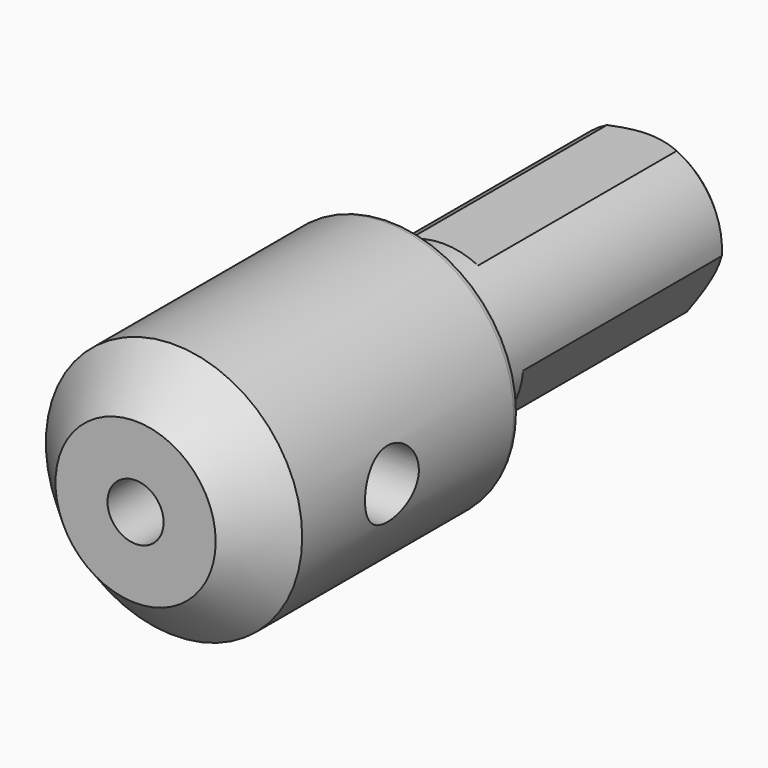
from build123d import *

# Parameters (mm, degrees)
F0_R            = 8
F1_DEPTH        = 20
F2_R            = 5
F3_DEPTH        = 20
F5_DEPTH        = 16
F5_COPIES_COUNT = 3
F6_SIZE         = 0.49999
F7_R            = 0.5
F9_D            = 3.5
F9_DEPTH        = 14
F9_TIP          = 1.0515060833
F10_R           = 2.1
F11_DEPTH       = 8.25
F12_SIZE        = 3


# Not quite as in the source:
# - a fillet or chamfer is up to 0.001 mm smaller than in the source, because OpenCascade refuses the exact size
# - a pattern or mirror of a feature is missing from the dataset's text; its kind, count and spacing are read off the source's solid


with BuildPart() as f1:
    # F0 (on Front) → F1 (new body)
    with BuildSketch(Plane.XZ):
        Circle(F0_R)
    extrude(amount=-F1_DEPTH)

    # F2 (on face) → F3 (join)
    with BuildSketch(Plane(origin=(0, 20, 0), x_dir=(-1, 0, 0), z_dir=(0, 1, 0))):
        Circle(F2_R)
    extrude(amount=F3_DEPTH)

    # F4 (on face) → F5 (cut)
    with BuildSketch(Plane(origin=(0, 40, 0), x_dir=(-1, 0, 0), z_dir=(0, 1, 0))):
        with BuildLine():
            ThreePointArc((2.1794494718, 4.5), (0, 5), (-2.1794494718, 4.5))
            Line((-2.1794494718, 4.5), (2.1794494718, 4.5))
        make_face()
    f5 = extrude(amount=-F5_DEPTH, mode=Mode.SUBTRACT)

    # F5_copies: F5 ×3 about axis
    f5_copies_axis = Axis((0, 0, 0), (0, 1, 0))
    for i in range(1, F5_COPIES_COUNT):
        add(f5.rotate(f5_copies_axis, i * 360 / F5_COPIES_COUNT), mode=Mode.SUBTRACT)

    # F6 (size 0.5 in the source; OpenCascade refuses exactly that, so slightly less here)
    f6_edges = [f1.edges().sort_by_distance(p)[0] for p in [
        (4.330127, 40, 2.5),
        (-4.996709, 40, -0.18139),
        (0, 40, -5),
        (-4.236582, 40, 2.655443),
    ]]
    chamfer(f6_edges, length=F6_SIZE)

    # F7
    f7_edges = [f1.edges().sort_by_distance(p)[0] for p in [
        (-8, 20, 0),
        (5, 20, 0),
    ]]
    fillet(f7_edges, radius=F7_R)

    # F9
    with Locations(Plane.XZ):
        with Locations((0, 0)):
            Hole(F9_D / 2, depth=F9_DEPTH)
            with Locations((0, 0, -(F9_DEPTH + F9_TIP / 2))):  # 118° drill point
                Cone(0, F9_D / 2, F9_TIP, mode=Mode.SUBTRACT)

    # F10 (on Right) → F11 (cut, symmetric)
    with BuildSketch(Plane.YZ):
        with Locations((10, 0)):
            Circle(F10_R)
    extrude(amount=F11_DEPTH, both=True, mode=Mode.SUBTRACT)

    # F12
    f12_edges = [f1.edges().sort_by_distance(p)[0] for p in [
        (-8, 0, 0),
    ]]
    chamfer(f12_edges, length=F12_SIZE)


solid = f1.part
